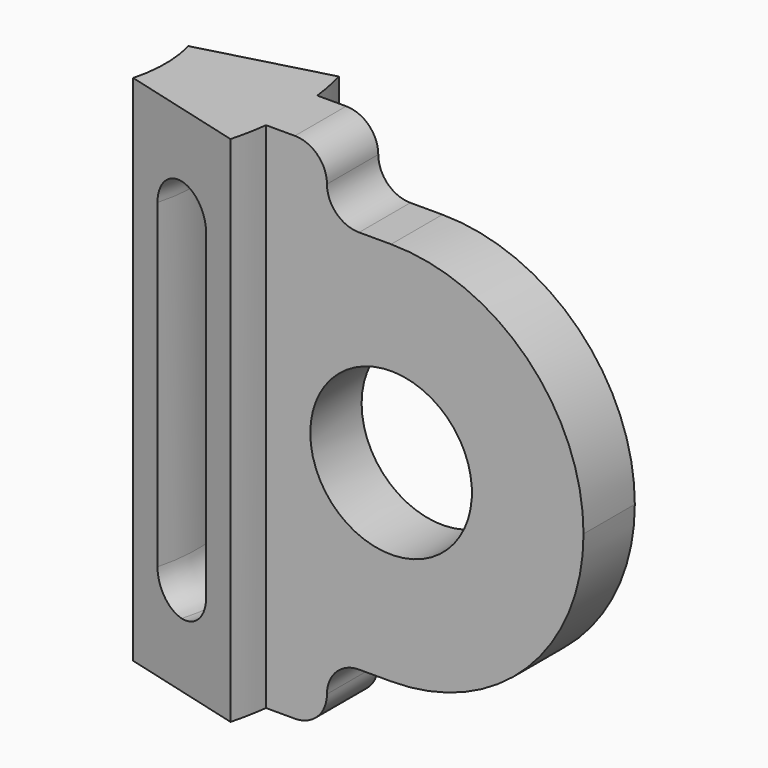
from build123d import *

# Parameters (mm, degrees)
F0_R      = 6.477
F0_R_2    = 3.302
F1_DEPTH  = 6.35
F3_DEPTH  = 0.79375
F4_R      = 0.79374
F5_R      = 4.76249
F7_D      = 4
F8_COUNT  = 12
F10_DEPTH = 12.701
F12_DEPTH = 4.7625
F13_R     = 0.79374


# Not quite as in the source:
# - a fillet or chamfer is up to 0.001 mm smaller than in the source, because OpenCascade refuses the exact size


with BuildPart() as f1:
    # F0 (on Top) → F1 (new body, symmetric)
    with BuildSketch(Plane.XY):
        Circle(F0_R)
        Circle(F0_R_2, mode=Mode.SUBTRACT)
    extrude(amount=F1_DEPTH, both=True)

    # F2 (on Front) → F3 (join, symmetric)
    with BuildSketch(Plane.XZ):
        Polygon((7.9375, 4.7625), (7.9375, 6.35), (4.7625, 6.35), (4.7625, -6.35), (7.9375, -6.35), (7.9375, -4.7625), (14.2875, -4.7625), (14.2875, 0), (14.2875, 4.7625), align=None)
    extrude(amount=F3_DEPTH, both=True)

    # F4 (radius 0.79375 in the source; OpenCascade refuses exactly that, so slightly less here)
    f4_edges = [f1.edges().sort_by_distance(p)[0] for p in [
        (7.9375, 0, 6.35),
        (7.9375, 0, 4.7625),
        (7.9375, 0, -6.35),
        (7.9375, 0, -4.7625),
    ]]
    fillet(f4_edges, radius=F4_R)

    # F5 (radius 4.7625 in the source; OpenCascade refuses exactly that, so slightly less here)
    f5_edges = [f1.edges().sort_by_distance(p)[0] for p in [
        (14.2875, 0, -4.7625),
        (14.2875, 0, 4.7625),
    ]]
    fillet(f5_edges, radius=F5_R)

    # F7 (through all)
    with Locations(Plane.XZ.offset(0.79375)):
        with Locations((9.525, 0)):
            Hole(F7_D / 2)

    # F8: F1 ×12 about axis
    f8_axis = Axis((0, 0, 6.35), (0, 0, 1))


with BuildPart() as f1_1:
    add(f1.part)
    for i in range(1, F8_COUNT):
        add(f1.part.rotate(f8_axis, i * 360 / F8_COUNT))

    # F9 (on face) → F10 (cut, through all)
    with BuildSketch(Plane.XY.offset(6.35)):
        with BuildLine():
            Line((3.1894870784, 0.8546204869), (6.2563015769, 1.6763709551))
            Line((6.2563015769, 1.6763709551), (15.3340724923, 4.108752341))
            ThreePointArc((15.3340724923, 4.108752341), (-15.875, 0), (15.3340724923, -4.108752341))
            Line((15.3340724923, -4.108752341), (6.2563015769, -1.6763709551))
            Line((6.2563015769, -1.6763709551), (3.1894870784, -0.8546204869))
            Line((3.1894870784, -0.8546204869), (3.1894870784, 0.8546204869))
        make_face()
    extrude(amount=-F10_DEPTH, mode=Mode.SUBTRACT)

    # F11 (on Top) → F12 (cut, symmetric)
    with BuildSketch(Plane.XY):
        with BuildLine():
            Line((3.956190703, -1.060058104), (4.7228943276, -1.265495721))
            Line((4.7228943276, -1.265495721), (5.4895979523, -1.4709333381))
            ThreePointArc((5.4895979523, -1.4709333381), (5.68325, 0), (5.4895979523, 1.4709333381))
            Line((5.4895979523, 1.4709333381), (4.7228943276, 1.265495721))
            Line((4.7228943276, 1.265495721), (3.956190703, 1.060058104))
            ThreePointArc((3.956190703, 1.060058104), (4.09575, 0), (3.956190703, -1.060058104))
        make_face()
    extrude(amount=F12_DEPTH, both=True, mode=Mode.SUBTRACT)

    # F13 (radius 0.79375 in the source; OpenCascade refuses exactly that, so slightly less here)
    f13_edges = [f1_1.edges().sort_by_distance(p)[0] for p in [
        (5.68325, 0, -4.7625),
        (4.09575, 0, -4.7625),
        (4.09575, 0, 4.7625),
        (5.68325, 0, 4.7625),
    ]]
    fillet(f13_edges, radius=F13_R)


solid = f1_1.part
